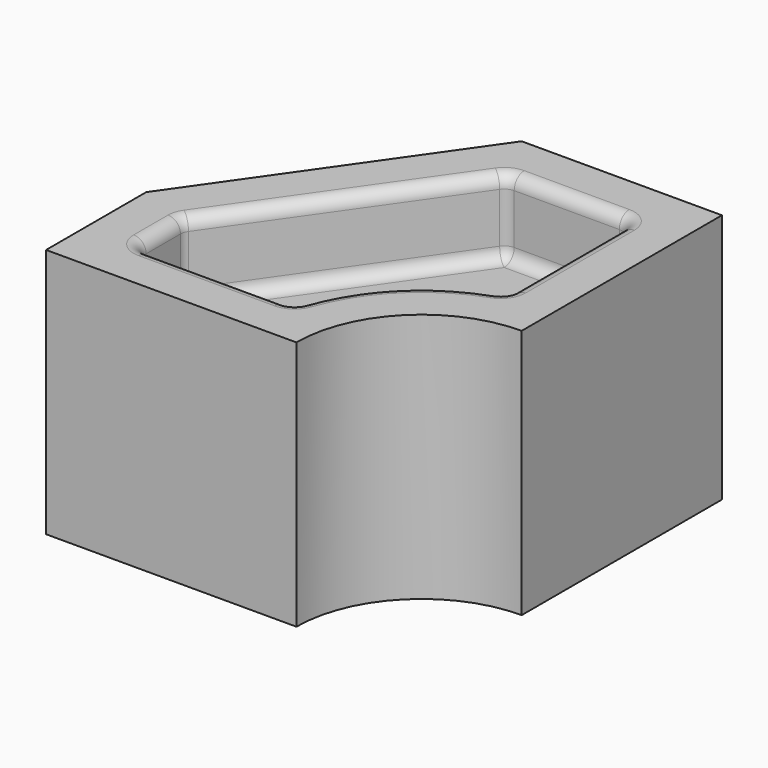
from build123d import *

# Parameters (mm, degrees)
F1_DEPTH = 100
F3_DEPTH = 30
F4_R     = 5


with BuildPart() as f1:
    # F0 (on Top) → F1 (new body)
    with BuildSketch(Plane.XY):
        with BuildLine():
            Line((0, 50), (0, 0))
            Line((0, 0), (100, 0))
            ThreePointArc((100, 0), (114.6446609407, 35.3553390593), (150, 50))
            Line((150, 50), (150, 150))
            Line((150, 150), (70, 150))
            Line((70, 150), (0, 50))
        make_face()
    extrude(amount=F1_DEPTH)

    # F2 (on face) → F3 (cut)
    with BuildSketch(Plane.XY.offset(100)):
        with BuildLine():
            Line((20, 43.6955553836), (20, 20))
            Line((20, 20), (82.917960675, 20))
            ThreePointArc((82.917960675, 20), (100.5025253169, 49.4974746831), (130, 67.082039325))
            Line((130, 67.082039325), (130, 130))
            Line((130, 130), (80.4131112315, 130))
            Line((80.4131112315, 130), (20, 43.6955553836))
        make_face()
    extrude(amount=-F3_DEPTH, mode=Mode.SUBTRACT)

    # F4
    f4_edges = [f1.edges().sort_by_distance(p)[0] for p in [
        (20, 31.847778, 70),
        (51.45898, 20, 70),
        (100.502525, 49.497475, 70),
        (130, 98.54102, 70),
        (105.206556, 130, 70),
        (50.206556, 86.847778, 70),
        (80.413111, 130, 85),
        (20, 43.695555, 85),
        (50.206556, 86.847778, 100),
        (82.917961, 20, 85),
        (130, 67.082039, 85),
        (100.502525, 49.497475, 100),
        (20, 20, 85),
        (20, 31.847778, 100),
        (130, 130, 85),
        (130, 98.54102, 100),
        (105.206556, 130, 100),
        (51.45898, 20, 100),
    ]]
    fillet(f4_edges, radius=F4_R)


solid = f1.part
